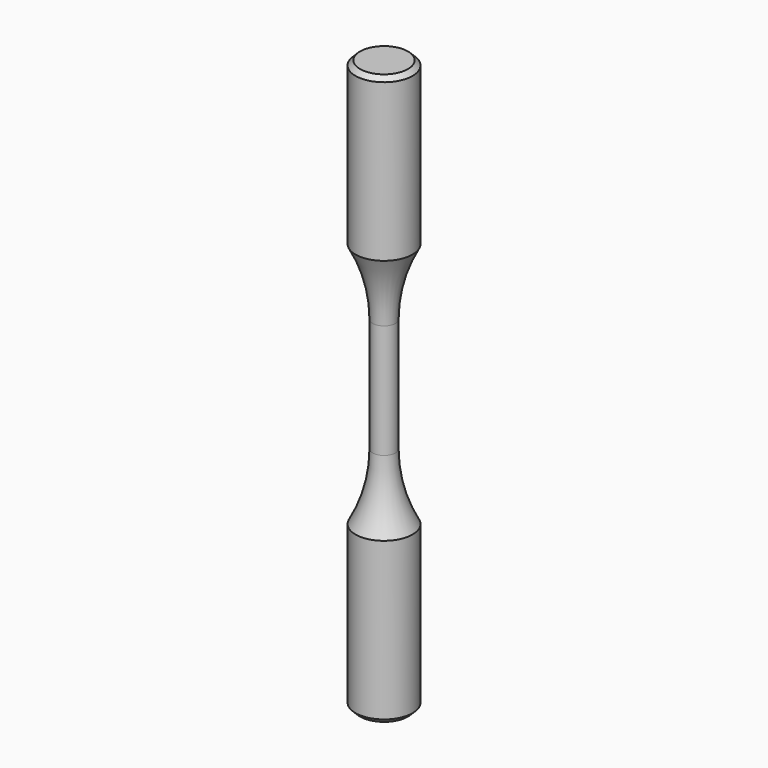
from build123d import *

# Parameters (mm, degrees)
F2_SIZE = 0.2


# Not quite as in the source:
# - a feature names something its author has since deleted; it is built from what else it names


with BuildPart() as f1:
    # F0 (on Front) → F1 (revolve)
    with BuildSketch(Plane.XZ):
        with BuildLine():
            Line((0, 12.5), (0, 0))
            Line((0, 0), (0, -12.5))
            Line((0, -12.5), (1.25, -12.5))
            Line((1.25, -12.5), (1.25, -5.4047375097))
            ThreePointArc((1.25, -5.4047375097), (0.6905249807, -4), (0.5, -2.5))
            Line((0.5, -2.5), (0.5, 0))
            Line((0.5, 0), (0.5, 2.5))
            ThreePointArc((0.5, 2.5), (0.6905249807, 4), (1.25, 5.4047375097))
            Line((1.25, 5.4047375097), (1.25, 12.5))
            Line((1.25, 12.5), (0, 12.5))
        make_face()
    revolve(axis=Axis((0, 0, 6.25), (0, 0, 1)))

    # F2
    f2_edges = [f1.edges().sort_by_distance(p)[0] for p in [
        (-1.25, 0, -12.5),
        (-1.25, 0, 12.5),
    ]]
    chamfer(f2_edges, length=F2_SIZE)


solid = f1.part
